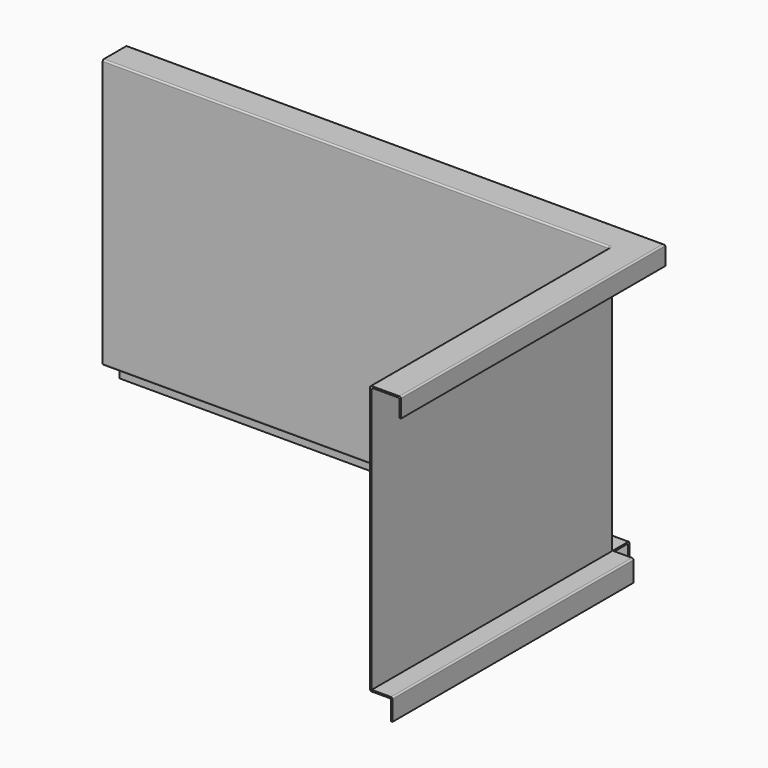
from build123d import *

# Parameters (mm, degrees)
F3_W         = 27
F3_H         = 27
F4_DEPTH     = 30
F5_T1_DEPTH  = 662
F5_T3_DEPTH  = 392
F5_T5_DEPTH  = 350
F5_T10_DEPTH = 433
F5_T15_DEPTH = 703
F5_T17_DEPTH = 402
F5_T19_DEPTH = 672
F5_T21_DEPTH = 710
F5_T23_DEPTH = 440
F5_T25_DEPTH = 346
F5_T27_DEPTH = 390
F5_T29_DEPTH = 660
F5_T32_ANGLE = 90
F5_T33_DEPTH = 393
F5_T35_DEPTH = 663
F5_T38_ANGLE = 90
F5_T40_ANGLE = 90


# Not quite as in the source:
# - a fillet or chamfer that OpenCascade refuses, or shapes differently, is made with other operations: its cross-section is extruded or revolved along the edge and cut away or added


with BuildPart() as f2:
    # F2: sweep along a path in F1
    with BuildLine(Plane.XY) as f2_path:
        Line((0, 0), (0, 390))
        Line((0, 390), (-660, 390))
    # F0 (on Front) → F2 (sweep)
    with BuildSketch(Plane.XZ):
        Polygon((38, -2), (38, -25), (40, -25), (40, 0), (0, 0), (0, -350), (27, -350), (27, -376), (29, -376), (29, -348), (2, -348), (2, -2), align=None)
    sweep(path=f2_path.line, transition=Transition.RIGHT)

    # F3 (on face) → F4 (cut)
    with BuildSketch(Plane.XY.offset(-348)):
        with Locations((15.5, 405.5)):
            Rectangle(F3_W, F3_H)
    extrude(amount=-F4_DEPTH, mode=Mode.SUBTRACT)

    # F5: fillet of radius 2 on 16 edges, made by hand

    # F5_s2 → F5_t1 (join)
    with BuildSketch(Plane.YZ.offset(-660)):
        with BuildLine():
            ThreePointArc((415, -350), (416.4142135624, -350.5857864376), (417, -352))
            Line((417, -352), (417, -350))
            Line((417, -350), (415, -350))
        make_face()
    extrude(amount=F5_T1_DEPTH)

    # F5_s4 → F5_t3 (join)
    with BuildSketch(Plane.XZ.offset(-392)):
        with BuildLine():
            ThreePointArc((25, -350), (26.4142135624, -350.5857864376), (27, -352))
            Line((27, -352), (27, -350))
            Line((27, -350), (25, -350))
        make_face()
    extrude(amount=F5_T3_DEPTH)

    # F5_s6 → F5_t5 (join)
    with BuildSketch(Plane.XY.offset(-350)):
        with BuildLine():
            ThreePointArc((0, 388), (-0.5857864376, 389.4142135624), (-2, 390))
            Line((-2, 390), (0, 390))
            Line((0, 390), (0, 388))
        make_face()
    extrude(amount=F5_T5_DEPTH)


with BuildPart() as f5_tool8:
    # F5_s9 → F5_t10 (new body)
    with BuildSketch(Plane.XZ):
        with BuildLine():
            ThreePointArc((38, -4), (37.4142135624, -2.5857864376), (36, -2))
            Line((36, -2), (38, -2))
            Line((38, -2), (38, -4))
        make_face()
    extrude(amount=-F5_T10_DEPTH)

    split(bisect_by=Plane.XZ.offset(-430), keep=Keep.TOP)


with BuildPart() as f2_1:
    add(f2.part)

    # F5_t7: union F5_tool8
    add(f5_tool8.part)


with BuildPart() as f5_tool13:
    # F5_s14 → F5_t15 (new body)
    with BuildSketch(Plane.YZ.offset(43)):
        with BuildLine():
            ThreePointArc((426, -2), (427.4142135624, -2.5857864376), (428, -4))
            Line((428, -4), (428, -2))
            Line((428, -2), (426, -2))
        make_face()
    extrude(amount=-F5_T15_DEPTH)

    split(bisect_by=Plane.YZ.offset(40), keep=Keep.BOTTOM)


with BuildPart() as f2_2:
    add(f2_1.part)

    # F5_t12: union F5_tool13
    add(f5_tool13.part)

    # F5_s18 → F5_t17 (cut)
    with BuildSketch(Plane.XZ.offset(-397)):
        with BuildLine():
            ThreePointArc((29, -350), (28.4142135624, -348.5857864376), (27, -348))
            Line((27, -348), (29, -348))
            Line((29, -348), (29, -350))
        make_face()
    extrude(amount=F5_T17_DEPTH, mode=Mode.SUBTRACT)

    # F5_s20 → F5_t19 (cut)
    with BuildSketch(Plane.YZ.offset(-665)):
        with BuildLine():
            ThreePointArc((419, -350), (418.4142135624, -348.5857864376), (417, -348))
            Line((417, -348), (419, -348))
            Line((419, -348), (419, -350))
        make_face()
    extrude(amount=F5_T19_DEPTH, mode=Mode.SUBTRACT)

    # F5_s22 → F5_t21 (cut)
    with BuildSketch(Plane.YZ.offset(-665)):
        with BuildLine():
            ThreePointArc((430, -2), (429.4142135624, -0.5857864376), (428, 0))
            Line((428, 0), (430, 0))
            Line((430, 0), (430, -2))
        make_face()
    extrude(amount=F5_T21_DEPTH, mode=Mode.SUBTRACT)

    # F5_s24 → F5_t23 (cut)
    with BuildSketch(Plane.XZ.offset(-435)):
        with BuildLine():
            ThreePointArc((40, -2), (39.4142135624, -0.5857864376), (38, 0))
            Line((38, 0), (40, 0))
            Line((40, 0), (40, -2))
        make_face()
    extrude(amount=F5_T23_DEPTH, mode=Mode.SUBTRACT)

    # F5_s26 → F5_t25 (cut)
    with BuildSketch(Plane.XY.offset(-348)):
        with BuildLine():
            ThreePointArc((2, 390), (1.4142135624, 391.4142135624), (0, 392))
            Line((0, 392), (2, 392))
            Line((2, 392), (2, 390))
        make_face()
    extrude(amount=F5_T25_DEPTH, mode=Mode.SUBTRACT)

    # F5_s28 → F5_t27 (join)
    with BuildSketch(Plane.XZ.offset(-390)):
        with BuildLine():
            ThreePointArc((4, -2), (2.5857864376, -2.5857864376), (2, -4))
            Line((2, -4), (2, -2))
            Line((2, -2), (4, -2))
        make_face()
    extrude(amount=F5_T27_DEPTH)

    # F5_s30 → F5_t29 (join)
    with BuildSketch(Plane.YZ.offset(-660)):
        with BuildLine():
            ThreePointArc((394, -2), (392.5857864376, -2.5857864376), (392, -4))
            Line((392, -4), (392, -2))
            Line((392, -2), (394, -2))
        make_face()
    extrude(amount=F5_T29_DEPTH)

    # F5_s31 → F5_t32 (revolve)
    with BuildSketch(Plane.XZ.offset(-390)):
        with BuildLine():
            ThreePointArc((4, -2), (2.5857864376, -2.5857864376), (2, -4))
            Line((2, -4), (2, -2))
            Line((2, -2), (4, -2))
        make_face()
    revolve(axis=Axis((0, 390, -2), (0, 0, 1)), revolution_arc=F5_T32_ANGLE)

    # F5_s34 → F5_t33 (cut)
    with BuildSketch(Plane.XZ.offset(-388)):
        with BuildLine():
            ThreePointArc((2, -350), (0.5857864376, -349.4142135624), (0, -348))
            Line((0, -348), (0, -350))
            Line((0, -350), (2, -350))
        make_face()
        with BuildLine():
            ThreePointArc((0, -2), (0.5857864376, -0.5857864376), (2, 0))
            Line((2, 0), (0, 0))
            Line((0, 0), (0, -2))
        make_face()
    extrude(amount=F5_T33_DEPTH, mode=Mode.SUBTRACT)

    # F5_s36 → F5_t35 (cut)
    with BuildSketch(Plane.YZ.offset(-665)):
        with BuildLine():
            ThreePointArc((392, -350), (390.5857864376, -349.4142135624), (390, -348))
            Line((390, -348), (390, -350))
            Line((390, -350), (392, -350))
        make_face()
        with BuildLine():
            ThreePointArc((392, 0), (390.5857864376, -0.5857864376), (390, -2))
            Line((390, -2), (390, 0))
            Line((390, 0), (392, 0))
        make_face()
    extrude(amount=F5_T35_DEPTH, mode=Mode.SUBTRACT)

    # F5_s37 → F5_t38 (revolve, cut)
    with BuildSketch(Plane.XZ.offset(-388)):
        with BuildLine():
            ThreePointArc((2, 0), (0.5857864376, -0.5857864376), (0, -2))
            Line((0, -2), (0, 0))
            Line((0, 0), (2, 0))
        make_face()
    revolve(axis=Axis((-2, 388, 0), (0, 0, 1)), revolution_arc=F5_T38_ANGLE, mode=Mode.SUBTRACT)

    # F5_s39 → F5_t40 (revolve, cut)
    with BuildSketch(Plane.XZ.offset(-388)):
        with BuildLine():
            ThreePointArc((2, -350), (0.5857864376, -349.4142135624), (0, -348))
            Line((0, -348), (0, -350))
            Line((0, -350), (2, -350))
        make_face()
    revolve(axis=Axis((-2, 388, -350), (0, 0, 1)), revolution_arc=F5_T40_ANGLE, mode=Mode.SUBTRACT)


solid = f2_2.part
